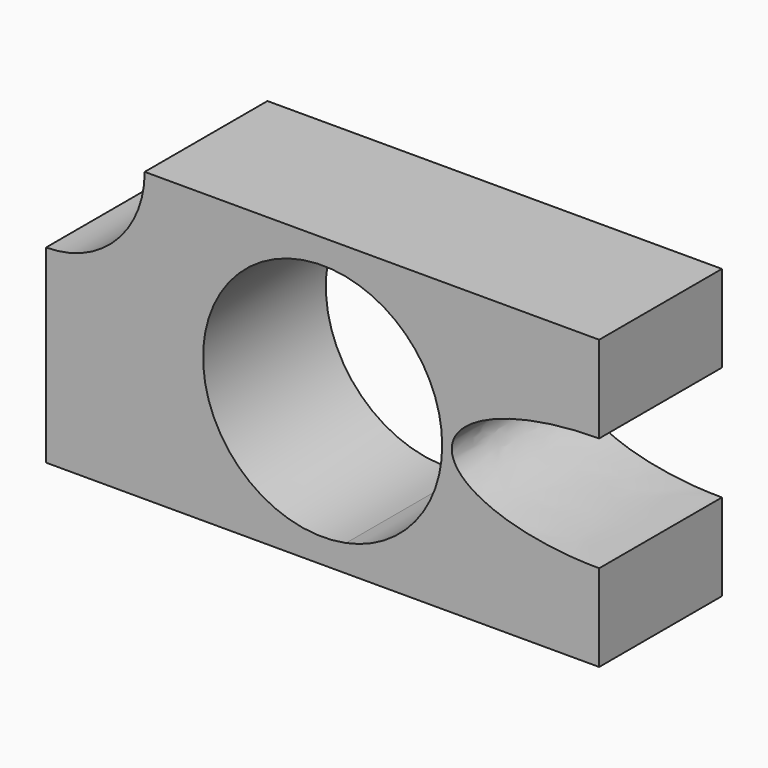
from build123d import *

# Parameters (mm, degrees)
F1_DEPTH = 25.4
F2_DEPTH = 25.4


with BuildPart() as f1:
    # F0 (on Front) → F1 (new body)
    with BuildSketch(Plane.XZ):
        with BuildLine():
            ThreePointArc((-29.4565436219, 23.8478247362), (-34.2387511178, 12.3025545416), (-45.7840213124, 7.5203470458))
            Line((-45.7840213124, 7.5203470458), (-45.7840213124, -23.8478247362))
            Line((-45.7840213124, -23.8478247362), (-3.5301e-06, -23.8478247362))
            ThreePointArc((-3.5301e-06, -23.8478247362), (2.0304351181, -21.7171458616), (3.8633102693, -19.4143123352))
            ThreePointArc((3.8633102693, -19.4143123352), (-19.7949662714, 0), (3.8633102693, 19.4143123352))
            ThreePointArc((3.8633102693, 19.4143123352), (2.0304351181, 21.7171458616), (-3.5301e-06, 23.8478247362))
            Line((-3.5301e-06, 23.8478247362), (-29.4565436219, 23.8478247362))
        make_face()
    extrude(amount=F1_DEPTH)

    # F0 (on Front) → F2 (join)
    with BuildSketch(Plane.XZ):
        with BuildLine():
            Line((45.7840142522, 23.8478247362), (-3.5301e-06, 23.8478247362))
            ThreePointArc((-3.5301e-06, 23.8478247362), (2.0304351181, 21.7171458616), (3.8633102693, 19.4143123352))
            ThreePointArc((3.8633102693, 19.4143123352), (15.3022022298, 12.5572009861), (19.7949662714, 0))
            ThreePointArc((19.7949662714, 0), (15.3022022298, -12.5572009861), (3.8633102693, -19.4143123352))
            ThreePointArc((3.8633102693, -19.4143123352), (2.0304351181, -21.7171458616), (-3.5301e-06, -23.8478247362))
            Line((-3.5301e-06, -23.8478247362), (45.7840283725, -23.8478247362))
            Line((45.7840283725, -23.8478247362), (45.7840241128, -9.4592027554))
            add(Edge.make_bspline(
                [(45.784018512, 9.4592027554), (21.3751961487, 9.4592016702), (21.3751989491, -1.0852e-06), (21.3752017495, -9.4592038407), (45.7840241128, -9.4592027554)],
                knots=[1.5707964415, 1.5707964415, 1.5707964415, 3.1415927683, 3.1415927683, 4.7123890951, 4.7123890951, 4.7123890951], degree=2, weights=[1, 0.7071067812, 1, 0.7071067812, 1]))
            Line((45.784018512, 9.4592027554), (45.7840142522, 23.8478247362))
        make_face()
    extrude(amount=F2_DEPTH)


solid = f1.part
